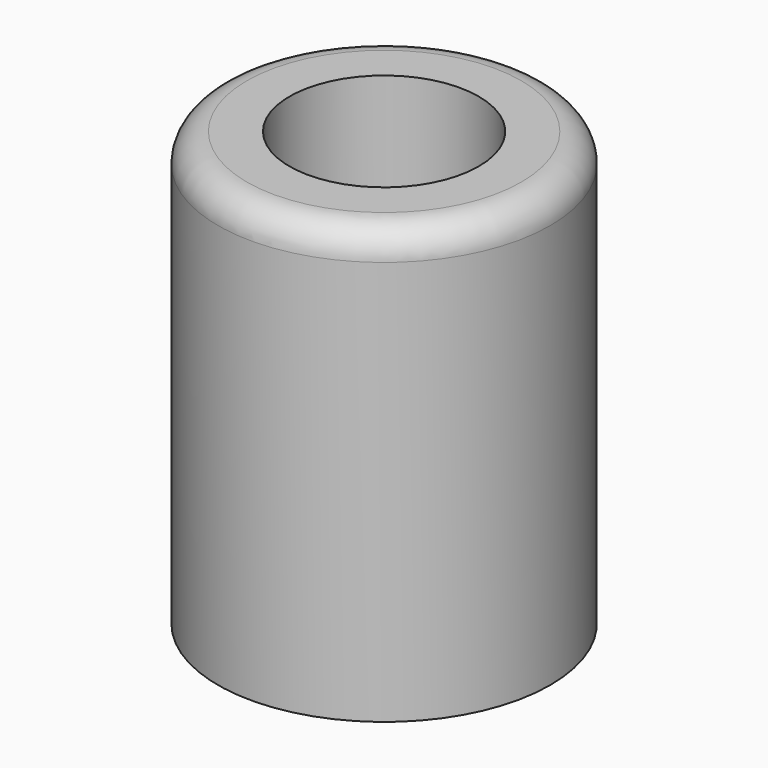
from build123d import *

# Parameters (mm, degrees)
F0_R         = 11.5
F1_DEPTH     = 30
F3_R         = 6.55
F4_DEPTH     = 25.3
F6_TEXT_SIZE = 6.3140144145
F7_DEPTH     = 3
F8_R         = 2


# Not quite as in the source:
# - Text() gives the source's letters only with a copy of the font that has no kerning and outlines rounded to 1/6400 em; it was checked with that copy


with BuildPart() as f1:
    # F0 (on Top) → F1 (new body)
    with BuildSketch(Plane.XY):
        Circle(F0_R)
    extrude(amount=F1_DEPTH)

    # F3 (on offset) → F4 (cut)
    with BuildSketch(Plane.XY.offset(30)):
        Circle(F3_R)
    extrude(amount=-F4_DEPTH, mode=Mode.SUBTRACT)

    # F6 (on offset) → F7 (cut)
    with BuildSketch(Plane(origin=(0, 0, 0), x_dir=(1, 0, 0), z_dir=(0, 0, -1))):
        with Locations((-5.8088940568, -1.3890831033)):
            Text('1/2', F6_TEXT_SIZE, font='Open Sans', font_style=FontStyle.BOLD, text_align=(TextAlign.LEFT, TextAlign.BOTTOM))
    extrude(amount=-F7_DEPTH, mode=Mode.SUBTRACT)

    # F8
    f8_edges = [f1.edges().sort_by_distance(p)[0] for p in [
        (-11.5, 0, 30),
    ]]
    fillet(f8_edges, radius=F8_R)


solid = f1.part
